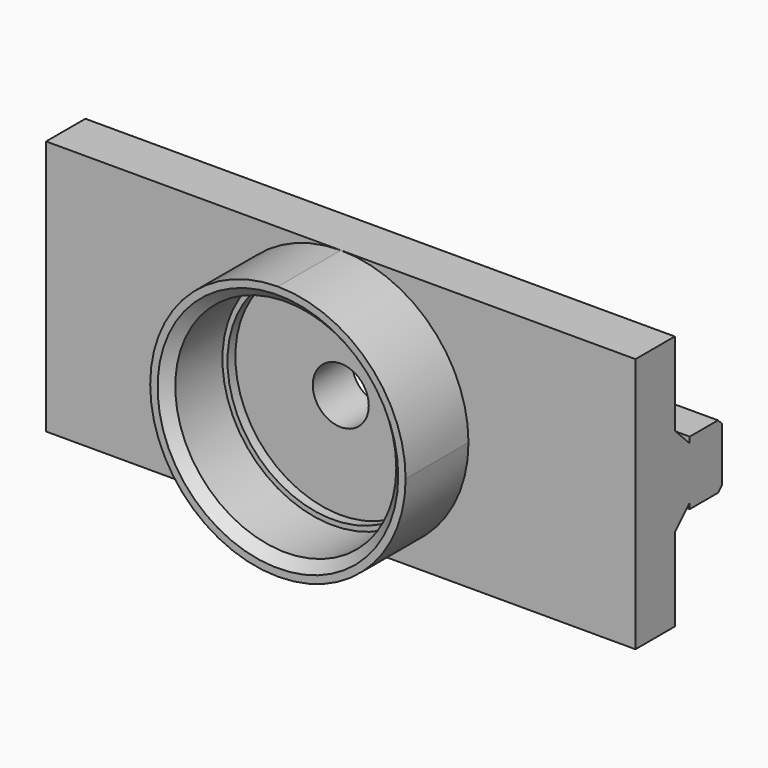
from build123d import *

# Parameters (mm, degrees)
F0_W        = 60
F0_H        = 26
F1_DEPTH    = 5
F2_R        = 11.25
F3_DEPTH    = 8
F4_R        = 11.25
F4_R_2      = 10.7332604818
F5_DEPTH    = 1
F6_SIZE     = 1
F7_W        = 60
F7_H        = 9.3
F8_DEPTH    = 1.9
F9_T4_DEPTH = 70.2867319519
F9_T9_DEPTH = 70.2867319519
F10_W       = 60
F10_H       = 6.5
F11_DEPTH   = 4.1
F12_SIZE    = 0.5
F13_R       = 2.85
F14_DEPTH   = 12.5
F15_W       = 6
F15_H       = 6
F16_DEPTH   = 12.5


# Not quite as in the source:
# - a fillet or chamfer that OpenCascade refuses, or shapes differently, is made with other operations: its cross-section is extruded or revolved along the edge and cut away or added


with BuildPart() as f1:
    # F0 (on Front) → F1 (new body)
    with BuildSketch(Plane.XZ):
        Rectangle(F0_W, F0_H)
    extrude(amount=F1_DEPTH)

    # F2 (on face) → F3 (join)
    with BuildSketch(Plane.XZ.offset(5)):
        with BuildLine():
            ThreePointArc((2.6e-08, -13), (9.1923881646, -9.1923881462), (13, 0))
            ThreePointArc((13, 0), (9.1923881562, 9.1923881546), (2.2e-09, 13))
            ThreePointArc((2.2e-09, 13), (-13, -1.19e-08), (2.6e-08, -13))
        make_face()
        Circle(F2_R, mode=Mode.SUBTRACT)
    extrude(amount=F3_DEPTH)

    # F4 (on face) → F5 (join)
    with BuildSketch(Plane.XZ.offset(5)):
        Circle(F4_R)
        Circle(F4_R_2, mode=Mode.SUBTRACT)
    extrude(amount=F5_DEPTH)

    # F6
    f6_edges = [f1.edges().sort_by_distance(p)[0] for p in [
        (-11.25, -13, 0),
    ]]
    chamfer(f6_edges, length=F6_SIZE)

    # F7 (on face) → F8 (join)
    with BuildSketch(Plane(origin=(0, 0, 0), x_dir=(-1, 0, 0), z_dir=(0, 1, 0))):
        Rectangle(F7_W, F7_H)
    extrude(amount=F8_DEPTH)

    # F9: chamfer of 2 on 2 edges, made by hand


with BuildPart() as f9_tool2:
    # F9_s3 → F9_t4 (new body)
    with BuildSketch(Plane.YZ.offset(-35.1433659759)):
        Polygon((-0.1, 4.65), (1.9, 2.65), (1.9, 4.65), align=None)
    extrude(amount=F9_T4_DEPTH)

    split(bisect_by=Plane.XZ, keep=Keep.BOTTOM)


with BuildPart() as f1_1:
    add(f1.part)

    # F9_t1: cut F9_tool2
    add(f9_tool2.part, mode=Mode.SUBTRACT)


with BuildPart() as f9_tool7:
    # F9_s8 → F9_t9 (new body)
    with BuildSketch(Plane.YZ.offset(35.1433659759)):
        Polygon((-0.1, -4.65), (1.9, -2.65), (1.9, -4.65), align=None)
    extrude(amount=-F9_T9_DEPTH)

    split(bisect_by=Plane.XZ, keep=Keep.BOTTOM)


with BuildPart() as f1_2:
    add(f1_1.part)

    # F9_t6: cut F9_tool7
    add(f9_tool7.part, mode=Mode.SUBTRACT)

    # F10 (on face) → F11 (join)
    with BuildSketch(Plane(origin=(0, 1.9, 0), x_dir=(-1, 0, 0), z_dir=(0, 1, 0))):
        Rectangle(F10_W, F10_H)
    extrude(amount=F11_DEPTH)

    # F12
    f12_edges = [f1_2.edges().sort_by_distance(p)[0] for p in [
        (0, 6, 3.25),
        (0, 6, -3.25),
    ]]
    chamfer(f12_edges, length=F12_SIZE)

    # F13 (on Front) → F14 (cut, symmetric)
    with BuildSketch(Plane.XZ):
        Circle(F13_R)
    extrude(amount=F14_DEPTH, both=True, mode=Mode.SUBTRACT)

    # F15 (on Top) → F16 (cut, symmetric)
    with BuildSketch(Plane.XY):
        with Locations((3, 3)):
            Rectangle(F15_W, F15_H)
        with Locations((-3, 3)):
            Rectangle(F15_W, F15_H)
    extrude(amount=F16_DEPTH, both=True, mode=Mode.SUBTRACT)


solid = f1_2.part
